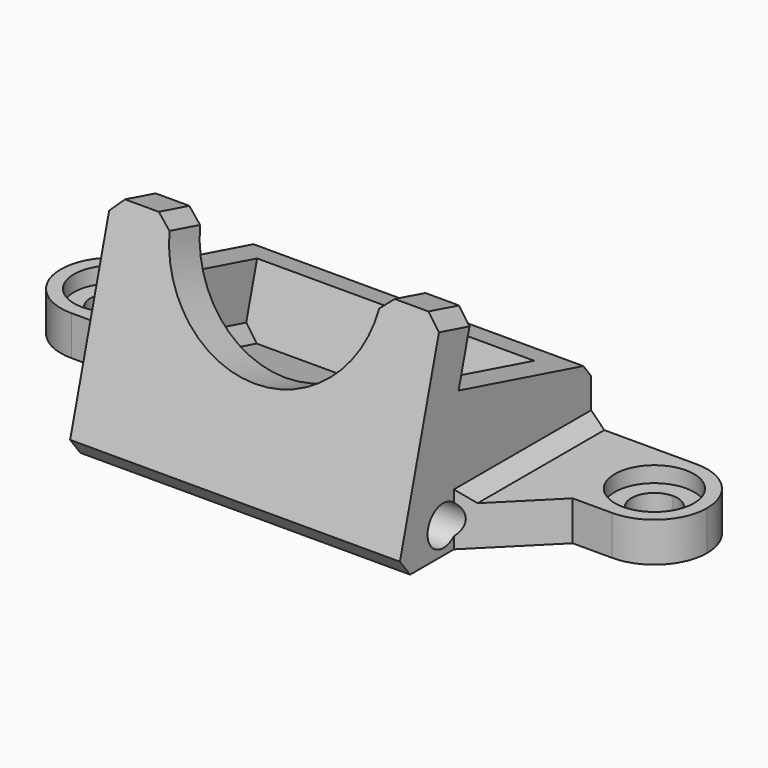
from build123d import *

# Parameters (mm, degrees)
F2_DEPTH       = 3
F3_R           = 3
F4_DEPTH       = 1.2
F5_DEPTH       = 12.5
F6_W           = 2
F6_H           = 10
F7_DEPTH       = 5
F9_DEPTH       = 3
F10_SIZE       = 5
F11_T1_DEPTH   = 15.1433659759
F11_T3_DEPTH   = 15.1433659759
F11_T5_DEPTH   = 8
F11_T10_DEPTH  = 7.571682988
F11_T15_DEPTH  = 7.571682988
F11_T17_DEPTH  = 7.8722554791
F11_T19_DEPTH  = 31.6397752967
F11_T21_DEPTH  = 8.1433659759
F11_T23_DEPTH  = 28.997160307
F12_R          = 1.5
F13_DEPTH      = 37.001
F13_DEPTH_BACK = 12.001


# Not quite as in the source:
# - a fillet or chamfer that OpenCascade refuses, or shapes differently, is made with other operations: its cross-section is extruded or revolved along the edge and cut away or added


with BuildPart() as f2:
    # F0 (on Top) → F2 (new body)
    with BuildSketch(Plane.XY):
        with BuildLine():
            ThreePointArc((20.5, -4), (16.5, 0), (20.5, 4))
            Line((20.5, 4), (-20.5, 4))
            ThreePointArc((-20.5, 4), (-17.6715728753, 2.8284271247), (-16.5, 0))
            ThreePointArc((-16.5, 0), (-17.6715728753, -2.8284271247), (-20.5, -4))
            Line((-20.5, -4), (20.5, -4))
        make_face()
        with BuildLine():
            ThreePointArc((24.5, 0), (23.3284271247, 2.8284271247), (20.5, 4))
            Line((20.5, 4), (20.5, 1.75))
            ThreePointArc((20.5, 1.75), (21.7374368671, 1.2374368671), (22.25, 0))
            ThreePointArc((22.25, 0), (21.7374368671, -1.2374368671), (20.5, -1.75))
            Line((20.5, -1.75), (20.5, -4))
            ThreePointArc((20.5, -4), (23.3284271247, -2.8284271247), (24.5, 0))
        make_face()
        with BuildLine():
            Line((20.5, 1.75), (20.5, 4))
            ThreePointArc((20.5, 4), (16.5, 0), (20.5, -4))
            Line((20.5, -4), (20.5, -1.75))
            ThreePointArc((20.5, -1.75), (18.75, 0), (20.5, 1.75))
        make_face()
        with BuildLine():
            ThreePointArc((-16.5, 0), (-17.6715728753, 2.8284271247), (-20.5, 4))
            Line((-20.5, 4), (-20.5, 1.75))
            ThreePointArc((-20.5, 1.75), (-19.2625631329, 1.2374368671), (-18.75, 0))
            ThreePointArc((-18.75, 0), (-19.2625631329, -1.2374368671), (-20.5, -1.75))
            Line((-20.5, -1.75), (-20.5, -4))
            ThreePointArc((-20.5, -4), (-17.6715728753, -2.8284271247), (-16.5, 0))
        make_face()
        with BuildLine():
            Line((-20.5, 1.75), (-20.5, 4))
            ThreePointArc((-20.5, 4), (-24.5, 0), (-20.5, -4))
            Line((-20.5, -4), (-20.5, -1.75))
            ThreePointArc((-20.5, -1.75), (-22.25, 0), (-20.5, 1.75))
        make_face()
    extrude(amount=F2_DEPTH)

    # F3 (on face) → F4 (cut)
    with BuildSketch(Plane.XY.offset(3)):
        with Locations((-20.5, 0)):
            Circle(F3_R)
        with Locations((20.5, 0)):
            Circle(F3_R)
    extrude(amount=-F4_DEPTH, mode=Mode.SUBTRACT)

    # F1 (on Right) → F5 (join, symmetric)
    with BuildSketch(Plane.YZ):
        Polygon((-14.454310627, 0), (0, 0), (4, 0), (4, 7.0531719961), (1.1022225211, 7.8296291314), (-0.1918727044, 3), (-9.8511309673, 5.588190451), (-7.2629405162, 15.2474487139), (-10.1607179951, 16.0239058492), align=None)
    extrude(amount=F5_DEPTH, both=True)

    # F6 (on face) → F7 (join, through all)
    with BuildSketch(Plane(origin=(0, 0.737146966, 2.7510699296), x_dir=(1, 0, 0), z_dir=(0, 0.2588190451, 0.9659258263))):
        with Locations((11.5, -5.9617919358)):
            Rectangle(F6_W, F6_H)
        with Locations((-11.5, -5.9617919358)):
            Rectangle(F6_W, F6_H)
    extrude(amount=F7_DEPTH)

    # F8 (on face) → F9 (cut, through all)
    with BuildSketch(Plane(origin=(0, -13.4860554121, 3.6135776568), x_dir=(1, 0, 0), z_dir=(0, -0.9659258263, 0.2588190451))):
        with BuildLine():
            ThreePointArc((-8, 12.8481171687), (0, 4.8481171687), (8, 12.8481171687))
            Line((8, 12.8481171687), (-8, 12.8481171687))
        make_face()
    extrude(amount=-F9_DEPTH, mode=Mode.SUBTRACT)

    # F10
    f10_edges = [f2.edges().sort_by_distance(p)[0] for p in [
        (-12.5, -4, 1.5),
        (12.5, -4, 1.5),
    ]]
    chamfer(f10_edges, length=F10_SIZE)

    # F11: chamfer of 1 on 12 edges, made by hand

    # F11_s2 → F11_t1 (join)
    with BuildSketch(Plane(origin=(0, -13.0723329483, 3.5027210567), x_dir=(1, 0, 0), z_dir=(0, 0.9659258263, -0.2588190451))):
        Polygon((-9.5, -2.8481171687), (-10.5, -3.8481171687), (-10.5, -2.8481171687), align=None)
    extrude(amount=F11_T1_DEPTH)

    # F11_s4 → F11_t3 (join)
    with BuildSketch(Plane(origin=(0, 1.5550353448, -0.4166704648), x_dir=(1, 0, 0), z_dir=(0, -0.9659258263, 0.2588190451))):
        Polygon((9.5, 2.8481171687), (10.5, 3.8481171687), (10.5, 2.8481171687), align=None)
    extrude(amount=F11_T3_DEPTH)

    # F11_s6 → F11_t5 (join)
    with BuildSketch(Plane.XZ.offset(-4)):
        Polygon((12.5, 4), (13.5, 3), (12.5, 3), align=None)
        Polygon((-13.5, 3), (-12.5, 4), (-12.5, 3), align=None)
    extrude(amount=F11_T5_DEPTH)


with BuildPart() as f11_tool8:
    # F11_s9 → F11_t10 (new body)
    with BuildSketch(Plane.XZ.offset(4)):
        Polygon((-13.5, 3), (-12.5, 4), (-12.5, 3), align=None)
    extrude(amount=F11_T10_DEPTH)

    split(bisect_by=Plane(origin=(-10.75, -10.75, 0), x_dir=(0, 0, 1), z_dir=(0.7071067812, 0.7071067812, 0)), keep=Keep.TOP)


with BuildPart() as f2_1:
    add(f2.part)

    # F11_t7: union F11_tool8
    add(f11_tool8.part)


with BuildPart() as f11_tool13:
    # F11_s14 → F11_t15 (new body)
    with BuildSketch(Plane.XZ.offset(4)):
        Polygon((12.5, 4), (13.5, 3), (12.5, 3), align=None)
    extrude(amount=F11_T15_DEPTH)

    split(bisect_by=Plane(origin=(10.75, -10.75, 0), x_dir=(0, 0, 1), z_dir=(-0.7071067812, 0.7071067812, 0)), keep=Keep.TOP)


with BuildPart() as f2_2:
    add(f2_1.part)

    # F11_t12: union F11_tool13
    add(f11_tool13.part)

    # F11_s18 → F11_t17 (cut)
    with BuildSketch(Plane(origin=(0, -15.8391741119, 4.244093912), x_dir=(1, 0, 0), z_dir=(0, 0.9659258263, -0.2588190451))):
        with BuildLine():
            Line((-7.95046392, -11.9592282798), (-8.94427191, -12.8481171687))
            Line((-8.94427191, -12.8481171687), (-8, -12.8481171687))
            ThreePointArc((-8, -12.8481171687), (-7.9868043053, -12.3888166251), (-7.95046392, -11.9592282798))
        make_face()
        with BuildLine():
            Line((8.94427191, -12.8481171687), (7.95046392, -11.9592282798))
            ThreePointArc((7.95046392, -11.9592282798), (7.9868043053, -12.3888166251), (8, -12.8481171687))
            Line((8, -12.8481171687), (8.94427191, -12.8481171687))
        make_face()
    extrude(amount=F11_T17_DEPTH, mode=Mode.SUBTRACT)

    # F11_s20 → F11_t19 (cut)
    with BuildSketch(Plane.YZ.offset(-15.8198876484)):
        Polygon((-14.1170110805, 1.2588190451), (-13.1510852542, 0), (-14.454310627, 0), align=None)
    extrude(amount=F11_T19_DEPTH, mode=Mode.SUBTRACT)

    # F11_s22 → F11_t21 (cut)
    with BuildSketch(Plane(origin=(0, -8.1042229181, 2.1715199862), x_dir=(1, 0, 0), z_dir=(0, -0.9659258263, 0.2588190451))):
        Polygon((-12.5, 11.8481171687), (-11.5, 12.8481171687), (-12.5, 12.8481171687), align=None)
        Polygon((11.5, 12.8481171687), (12.5, 11.8481171687), (12.5, 12.8481171687), align=None)
    extrude(amount=F11_T21_DEPTH, mode=Mode.SUBTRACT)

    # F11_s24 → F11_t23 (cut)
    with BuildSketch(Plane.YZ.offset(-14.4985801535)):
        Polygon((4, 6.2858450082), (3.2588190451, 7.2517708344), (4, 7.0531719961), align=None)
    extrude(amount=F11_T23_DEPTH, mode=Mode.SUBTRACT)

    # F12 (on face) → F13 (cut, two sides)
    with BuildSketch(Plane(origin=(-12.5, 0, 0), x_dir=(0, -1, 0), z_dir=(-1, 0, 0))) as f13_sk:
        with Locations((10, 2)):
            Circle(F12_R)
    extrude(amount=-F13_DEPTH, mode=Mode.SUBTRACT)
    extrude(f13_sk.sketch, amount=F13_DEPTH_BACK, mode=Mode.SUBTRACT)


solid = f2_2.part
